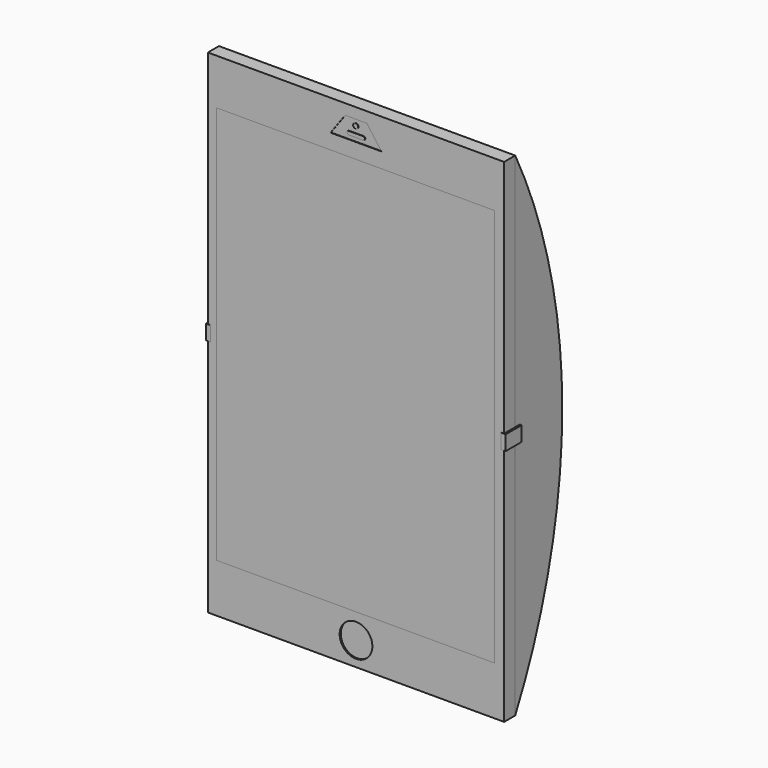
from build123d import *

# Parameters (mm, degrees)
F1_DEPTH  = 3.81
F2_W      = 76.4005258679
F2_H      = 109.6077784896
F3_DEPTH  = 0.254
F4_W      = 76.4005258679
F4_H      = 109.6077784896
F5_DEPTH  = 0.254
F6_R      = 0.6800962697
F7_DEPTH  = 0.127
F8_DEPTH  = 0.127
F9_DEPTH  = 0.127
F2_R      = 4.4974633364
F10_DEPTH = 0.381
F12_DEPTH = 81.5139375627
F14_DEPTH = 0.127
F15_W     = 3.81
F15_H     = 4.064
F16_DEPTH = 0.508
F17_W     = 0.1016
F17_H     = 4.064
F18_DEPTH = 1.27
F20_DEPTH = 0.508
F21_W     = 0.1016
F21_H     = 4.064
F22_DEPTH = 1.27


with BuildPart() as f1:
    # F0 (on Front) → F1 (new body)
    with BuildSketch(Plane.XZ):
        Polygon((-40.7569687814, -67.5272345543), (0, -67.5272345543), (40.7569687814, -67.5272345543), (40.7569687814, 68.1288167834), (0, 68.1288167834), (-40.7569687814, 68.1288167834), align=None)
    extrude(amount=F1_DEPTH)

    # F2 (on face) → F3 (cut)
    with BuildSketch(Plane.XZ.offset(3.81)):
        with Locations((-0.1503936946, 0.691767782)):
            Rectangle(F2_W, F2_H)
    extrude(amount=-F3_DEPTH, mode=Mode.SUBTRACT)

    # F6 (on face) → F7 (cut)
    with BuildSketch(Plane.XZ.offset(3.81)):
        Polygon((2.9781554878, 65.2042552829), (0, 65.2042552829), (-2.9781554878, 65.2042552829), (-7.0130091316, 59.6828758717), (0, 59.6828758717), (7.0130091316, 59.6828758717), align=None)
        with Locations((0, 63.6167749763)):
            Circle(F6_R, mode=Mode.SUBTRACT)
    extrude(amount=-F7_DEPTH, mode=Mode.SUBTRACT)

    # F8 (cut): a face of the model
    f8_faces = [f1.faces().sort_by_distance(p)[0] for p in [
        (0, -3.81, 63.6167749763),
    ]]
    extrude(f8_faces, amount=-F8_DEPTH, mode=Mode.SUBTRACT)

    # F2 (on face) → F10 (cut)
    with BuildSketch(Plane.XZ.offset(3.81)):
        with Locations((0, -61.009131372)):
            Circle(F2_R)
    extrude(amount=-F10_DEPTH, mode=Mode.SUBTRACT)

    # F13 (on face) → F14 (join)
    with BuildSketch(Plane.XZ.offset(3.683)):
        with BuildLine():
            Line((1.9728252664, 61.7312639952), (0, 61.7312639952))
            Line((0, 61.7312639952), (-1.9728252664, 61.7312639952))
            ThreePointArc((-1.9728252664, 61.7312639952), (-2.4538422003, 61.2502470613), (-1.9728252664, 60.7692301273))
            Line((-1.9728252664, 60.7692301273), (0, 60.7692301273))
            Line((0, 60.7692301273), (1.9728252664, 60.7692301273))
            ThreePointArc((1.9728252664, 60.7692301273), (2.4538422003, 61.2502470613), (1.9728252664, 61.7312639952))
        make_face()
    extrude(amount=F14_DEPTH)


with BuildPart() as f5:
    # F4 (on face) → F5 (new body)
    with BuildSketch(Plane.XZ.offset(3.556)):
        with Locations((-0.1503936946, 0.691767782)):
            Rectangle(F4_W, F4_H)
    extrude(amount=F5_DEPTH)


with BuildPart() as f9:
    # F6 (on face) → F9 (new body)
    with BuildSketch(Plane.XZ.offset(3.81)):
        with Locations((0, 63.6167749763)):
            Circle(F6_R)
    extrude(amount=F9_DEPTH)


with BuildPart() as f12:
    # F11 (on face) → F12 (new body, through all)
    with BuildSketch(Plane.YZ.offset(40.7569687814)):
        with BuildLine():
            Line((0, 68.1288167834), (0, -67.5272345543))
            ThreePointArc((0, -67.5272345543), (16.1784054614, 0.3007911146), (0, 68.1288167834))
        make_face()
    extrude(amount=-F12_DEPTH)

    # F15 (on face) → F16 (join)
    with BuildSketch(Plane.YZ.offset(40.7569687814)):
        with Locations((-1.905, 0.3007911146)):
            Rectangle(F15_W, F15_H)
        Polygon((1.5467249905, -1.7312088854), (1.5467249905, 0.3007911146), (1.5467249905, 2.3327911146), (0, 2.3327911146), (0, -1.7312088854), align=None)
    extrude(amount=F16_DEPTH)

    # F17 (on face) → F18 (join)
    with BuildSketch(Plane.YZ.offset(41.2649687814)):
        with Locations((-3.8608, 0.3007911146)):
            Rectangle(F17_W, F17_H)
    extrude(amount=-F18_DEPTH)

    # F19 (on face) → F20 (join)
    with BuildSketch(Plane(origin=(-40.7569687814, 0, 0), x_dir=(0, -1, 0), z_dir=(-1, 0, 0))):
        Polygon((0, -1.7312088854), (0, 2.3327911146), (-1.778, 2.3327911146), (-1.778, 0.3007911146), (-1.778, -1.7312088854), align=None)
        Polygon((3.81, -1.7312088854), (3.81, 0.3007911146), (3.81, 2.3327911146), (0, 2.3327911146), (0, -1.7312088854), align=None)
    extrude(amount=F20_DEPTH)

    # F21 (on face) → F22 (join)
    with BuildSketch(Plane(origin=(-41.2649687814, 0, 0), x_dir=(0, -1, 0), z_dir=(-1, 0, 0))):
        with Locations((3.8608, 0.3007911146)):
            Rectangle(F21_W, F21_H)
    extrude(amount=-F22_DEPTH)


solid = Compound([f1.part, f5.part, f9.part, f12.part])
